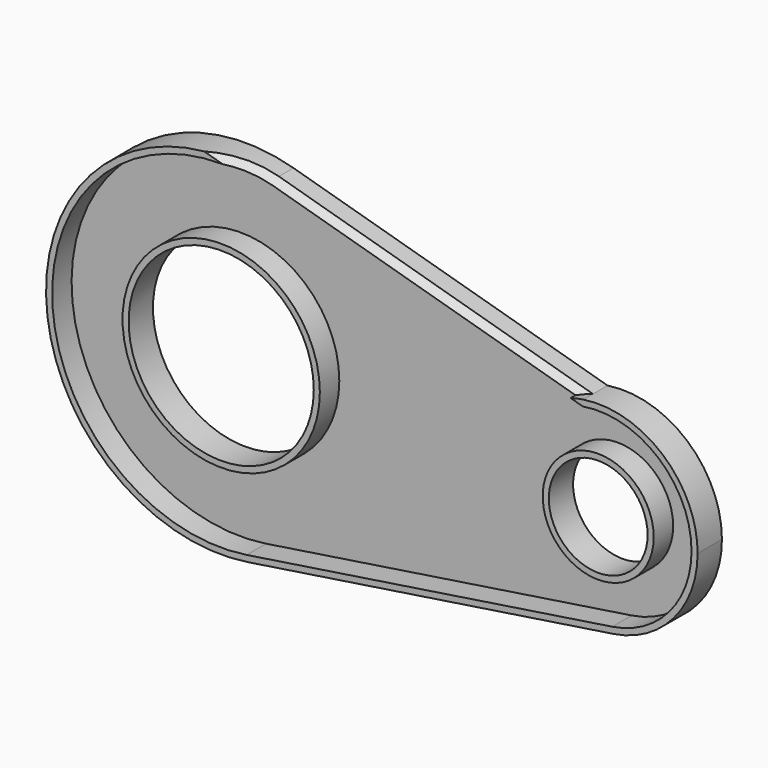
from build123d import *

# Parameters (mm, degrees)
F0_R        = 38.6786134899
F0_R_2      = 20.6427828865
F1_DEPTH    = 12.7
F2_T        = -2.54
F3_T4_DEPTH = 240.9522929605
F3_S5_R     = 41.5273672124
F3_T6_DEPTH = 123


# Not quite as in the source:
# - a fillet or chamfer that OpenCascade refuses, or shapes differently, is made with other operations: its cross-section is extruded or revolved along the edge and cut away or added


with BuildPart() as f1:
    # F0 (on Front) → F1 (new body)
    with BuildSketch(Plane.XZ):
        with BuildLine():
            ThreePointArc((-94.9406012258, -72.3378666508), (-50.4602870277, -47.6856781771), (-32.7881381913, 0))
            ThreePointArc((-32.7881381913, 0), (-47.5673995621, 44.0958373502), (-85.9349974728, 70.3788521857))
            ThreePointArc((-85.9349974728, 70.3788521857), (-178.9877879079, 4.6081079803), (-94.9406012258, -72.3378666508))
        make_face()
        with Locations((-105.9605851769, 0)):
            Circle(F0_R, mode=Mode.SUBTRACT)
        with BuildLine():
            ThreePointArc((-85.9349974728, 70.3788521857), (-47.5673995621, 44.0958373502), (-32.7881381913, 0))
            ThreePointArc((-32.7881381913, 0), (-50.4602870277, -47.6856781771), (-94.9406012258, -72.3378666508))
            Line((-94.9406012258, -72.3378666508), (57.8033803815, -49.0687780824))
            ThreePointArc((57.8033803815, -49.0687780824), (10.4955177286, -14.2692006943), (45.2950951166, 33.0386619586))
            Line((45.2950951166, 33.0386619586), (-85.9349974728, 70.3788521857))
        make_face()
        with BuildLine():
            ThreePointArc((93.0766049614, -8.0150580619), (78.6121658048, 23.4828808015), (45.2950951166, 33.0386619586))
            ThreePointArc((45.2950951166, 33.0386619586), (10.4955177286, -14.2692006943), (57.8033803815, -49.0687780824))
            ThreePointArc((57.8033803815, -49.0687780824), (83.0471766125, -35.0779861176), (93.0766049614, -8.0150580619))
        make_face()
        with Locations((51.5492377491, -8.0150580619)):
            Circle(F0_R_2, mode=Mode.SUBTRACT)
    extrude(amount=F1_DEPTH)

    # F2
    f2_openings = [f1.faces().sort_by_distance(p)[0] for p in [
        (-50.29361, -12.7, -3.378795),
    ]]
    offset(amount=F2_T, openings=f2_openings, kind=Kind.INTERSECTION)

    # F3: chamfer of 5.08 on 1 edges, made by hand


with BuildPart() as f3_tool2:
    # F3_s3 → F3_t4 (new body)
    with BuildSketch(Plane(origin=(96.0327547633, 0, -27.3251451716), x_dir=(0, 1, 0), z_dir=(-0.961821766, 0, 0.2736766164))):
        Polygon((-7.62, -44.1735125635), (-12.7, -39.0935125635), (-12.7, -44.1735125635), align=None)
    extrude(amount=F3_T4_DEPTH)

    # F3_s5 → F3_t6 (cut, symmetric)
    with BuildSketch(Plane.XZ.offset(10.2)):
        with Locations((51.5492377491, -8.0150580619)):
            Circle(F3_S5_R)
    extrude(amount=F3_T6_DEPTH, both=True, mode=Mode.SUBTRACT)


with BuildPart() as f1_1:
    add(f1.part)

    # F3_t1: cut F3_tool2
    add(f3_tool2.part, mode=Mode.SUBTRACT)


solid = f1_1.part
